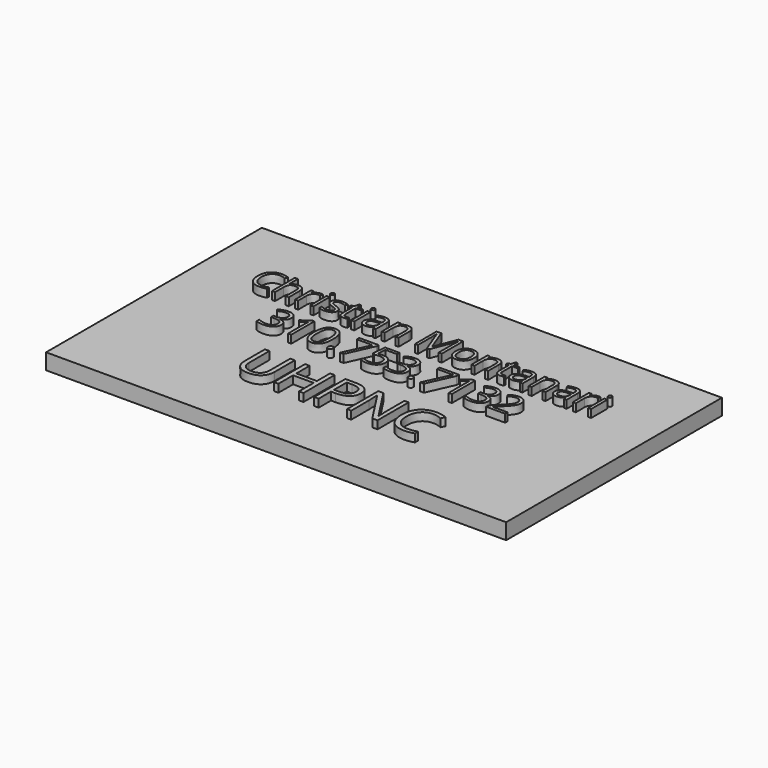
from build123d import *

# Parameters (mm, degrees)
F0_W           = 92.075
F0_H           = 53.975
F1_DEPTH       = 3.175
F2_TEXT_SIZE   = 7.5382358397
F2_TEXT_SIZE_2 = 8.1142058501
F2_TEXT_SIZE_3 = 10.9242417454
F3_DEPTH       = 1.5875


# Not quite as in the source:
# - Text() gives the source's letters only with a copy of the font that has no kerning and outlines rounded to 1/6400 em; it was checked with that copy


with BuildPart() as f1:
    # F0 (on Top) → F1 (new body)
    with BuildSketch(Plane.XY):
        with Locations((-46.0375, 26.9875)):
            Rectangle(F0_W, F0_H)
    extrude(amount=F1_DEPTH)

    # F2 (on face) → F3 (join)
    with BuildSketch(Plane.XY.offset(3.175)):
        with Locations((-80.9625, 35.8474701954)):
            Text('Christian Montanari', F2_TEXT_SIZE, font='Open Sans', text_align=(TextAlign.LEFT, TextAlign.BOTTOM))
        with Locations((-71.4375, 26.1952419834)):
            Text('310.753.7132', F2_TEXT_SIZE_2, font='Open Sans', text_align=(TextAlign.LEFT, TextAlign.BOTTOM))
        with Locations((-65.0875, 11.9797879267)):
            Text('UHPNC', F2_TEXT_SIZE_3, font='Open Sans', text_align=(TextAlign.LEFT, TextAlign.BOTTOM))
    extrude(amount=F3_DEPTH)


solid = f1.part
